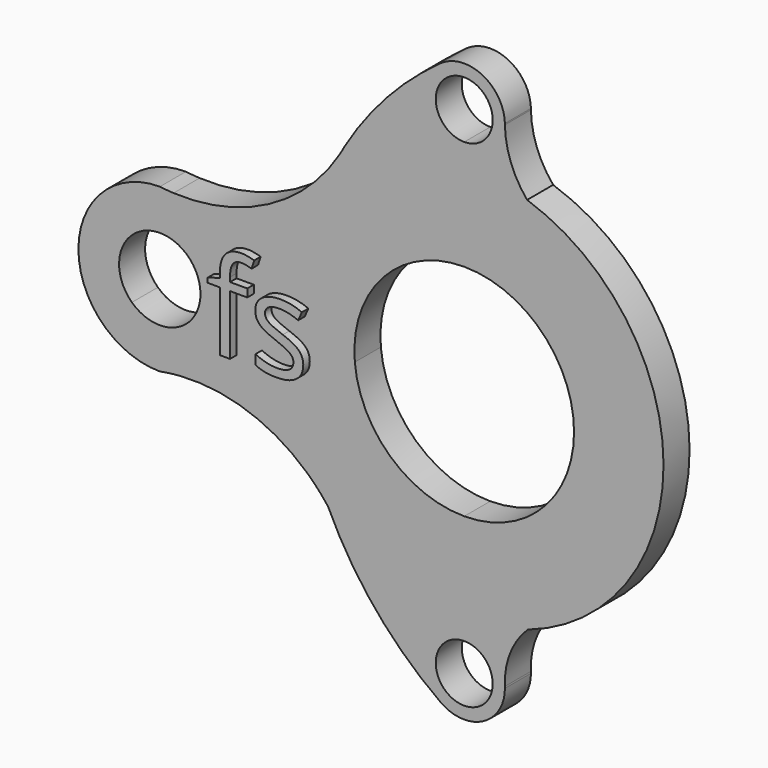
from build123d import *

# Parameters (mm, degrees)
F1_DEPTH     = 8
F2_TEXT_SIZE = 31.0813865831
F3_DEPTH     = 2


# Not quite as in the source:
# - Text() gives the source's letters only with a copy of the font that has no kerning and outlines rounded to 1/6400 em; it was checked with that copy


with BuildPart() as f1:
    # F0 (on Front) → F1 (new body)
    with BuildSketch(Plane.XZ):
        with BuildLine():
            ThreePointArc((-26.8935179321, -2.3955569786), (-19.9208438378, 18.2252566728), (0, 27))
            Line((0, 27), (0, 51))
            ThreePointArc((0, 51), (-9.5219045714, 57.9449495367), (-5.8179797945, 69.1333333333))
            ThreePointArc((-5.8179797945, 69.1333333333), (-18.9623337312, 57.5029806349), (-29.4378458081, 43.4209782549))
            ThreePointArc((-29.4378458081, 43.4209782549), (-30.0392798596, 42.3405233834), (-30.6700361416, 41.2769199985))
            ThreePointArc((-30.6700361416, 41.2769199985), (-48.0985934629, 24.9031610367), (-71.4412391919, 19.7093682793))
            ThreePointArc((-71.4412391919, 19.7093682793), (-73.1277073744, 19.8231941961), (-74.8087424009, 19.9999779887))
            ThreePointArc((-74.8087424009, 19.9999779887), (-94.8384043669, 0.0204169538), (-74.849576304, -19.9999968855))
            ThreePointArc((-74.849576304, -19.9999968855), (-72.2900400666, -19.5862442644), (-69.7098458461, -19.3312643303))
            ThreePointArc((-69.7098458461, -19.3312643303), (-53.0494604112, -21.5761696578), (-38.6051852955, -30.1768067943))
            ThreePointArc((-38.6051852955, -30.1768067943), (-35.904557685, -32.8701783), (-33.4594951415, -35.7975164624))
            ThreePointArc((-33.4594951415, -35.7975164624), (-21.797298439, -54.2552684297), (-5.8179797945, -69.1333333333))
            ThreePointArc((-5.8179797945, -69.1333333333), (-9.5219045714, -57.9449495367), (0, -51))
            Line((0, -51), (0, -27))
            ThreePointArc((0, -27), (-18.2252566728, -19.9208438378), (-26.8935179321, -2.3955569786))
        make_face()
        with BuildLine():
            ThreePointArc((-64.8384147882, 0), (-65.341842882, -3.132909515), (-66.801439194, -5.950380097))
            ThreePointArc((-66.801439194, -5.950380097), (-73.9511714628, -9.9605621971), (-81.6971333046, -7.2772233931))
            ThreePointArc((-81.6971333046, -7.2772233931), (-78.8015458002, 9.1811542075), (-64.8384147882, 0))
        make_face(mode=Mode.SUBTRACT)
        with BuildLine():
            ThreePointArc((0, 27), (19.091883092, 19.091883092), (27, 0))
            ThreePointArc((27, 0), (19.091883092, -19.091883092), (0, -27))
            Line((0, -27), (0, -51))
            ThreePointArc((0, -51), (6.9173900534, -53.7785240533), (9.990753177, -60.5700570303))
            ThreePointArc((9.990753177, -60.5700570303), (11.2967917868, -52.9024451031), (15.6270969838, -46.4412945541))
            ThreePointArc((15.6270969838, -46.4412945541), (48.9999248096, 0.0858408599), (15.4642845529, 46.4957622076))
            ThreePointArc((15.4642845529, 46.4957622076), (11.4789955325, 53.253493516), (9.9999124401, 60.95815277))
            ThreePointArc((9.9999124401, 60.95815277), (7.0562570708, 53.9141524042), (0, 51))
            Line((0, 51), (0, 27))
        make_face()
        with BuildLine():
            ThreePointArc((-5.8179797945, 69.1333333333), (-9.5219045714, 57.9449495367), (0, 51))
            ThreePointArc((0, 51), (7.0562570708, 53.9141524042), (9.9999124401, 60.95815277))
            ThreePointArc((9.9999124401, 60.95815277), (9.9976321382, 61.1132418295), (9.9963989601, 61.2683427497))
            ThreePointArc((9.9963989601, 61.2683427497), (4.4530120032, 69.9538083573), (-5.8179797945, 69.1333333333))
        make_face()
        with BuildLine():
            ThreePointArc((7, 61), (4.9497474683, 56.0502525317), (0, 54))
            ThreePointArc((0, 54), (-4.9497474683, 65.9497474683), (7, 61))
        make_face(mode=Mode.SUBTRACT)
        with BuildLine():
            ThreePointArc((9.990753177, -60.5700570303), (6.9173900534, -53.7785240533), (0, -51))
            ThreePointArc((0, -51), (-9.5219045714, -57.9449495367), (-5.8179797945, -69.1333333333))
            ThreePointArc((-5.8179797945, -69.1333333333), (4.5727563928, -69.8932501917), (10, -61))
            ThreePointArc((10, -61), (9.997688027, -60.7849788028), (9.990753177, -60.5700570303))
        make_face()
        with BuildLine():
            ThreePointArc((7, -61), (-4.9497474683, -65.9497474683), (0, -54))
            ThreePointArc((0, -54), (4.9497474683, -56.0502525317), (7, -61))
        make_face(mode=Mode.SUBTRACT)
    extrude(amount=F1_DEPTH)

    # F2 (on face) → F3 (join)
    with BuildSketch(Plane.XZ.offset(8)):
        with Locations((-61.8998743594, -10.3394789621)):
            Text('fs', F2_TEXT_SIZE, font='Open Sans', text_align=(TextAlign.LEFT, TextAlign.BOTTOM))
    extrude(amount=F3_DEPTH)


solid = f1.part
